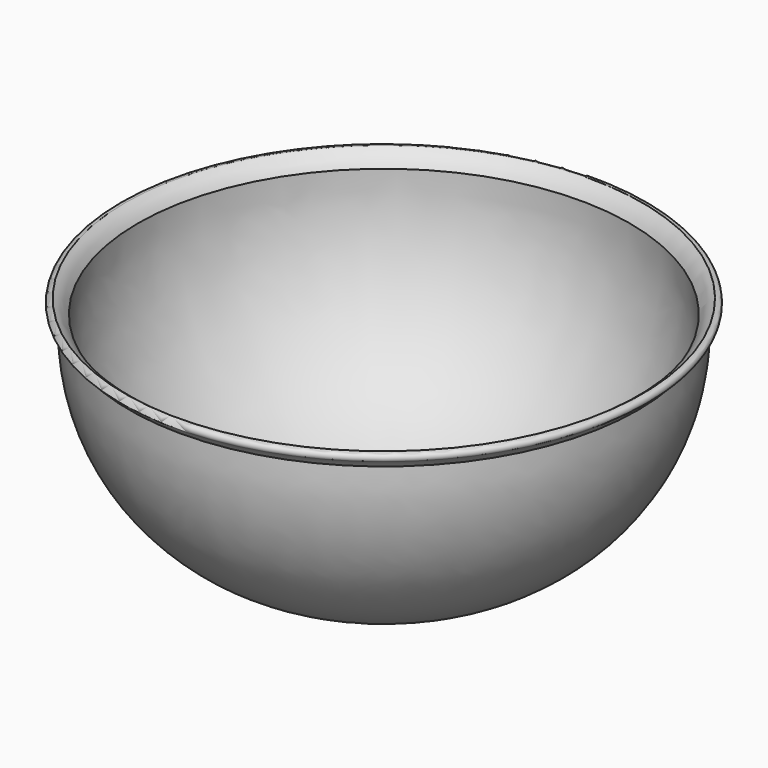
from build123d import *

# Parameters (mm, degrees)
F2_TEXT_SIZE = 18.1491480261
F3_DEPTH     = 3.175


# Not quite as in the source:
# - Text() gives the source's letters only with a copy of the font that has no kerning and outlines rounded to 1/6400 em; it was checked with that copy


with BuildPart() as f1:
    # F0 (on Front) → F1 (revolve)
    with BuildSketch(Plane.XZ):
        with BuildLine():
            ThreePointArc((0, 0), (-34.2352394172, 31.1750034287), (-45.0371901893, 76.2))
            ThreePointArc((-45.0371901893, 76.2), (-47.0998938701, 79.2854492393), (-49.9665268701, 81.6428119026))
            ThreePointArc((-49.9665268701, 81.6428119026), (-51.8145206739, 80.9019000279), (-51.6031930226, 78.9221596084))
            ThreePointArc((-51.6031930226, 78.9221596084), (-49.7126642737, 77.4294196755), (-48.2570643, 75.5101489353))
            ThreePointArc((-48.2570643, 75.5101489353), (-36.5560461644, 28.8693888765), (-0.7031318367, -3.175))
            Line((-0.7031318367, -3.175), (50.8, -3.175))
            Line((50.8, -3.175), (50.8, 0))
            Line((50.8, 0), (0, 0))
        make_face()
    revolve(axis=Axis((50.8, 0, -1.5875), (0, 0, 1)))

    # F2 (on face) → F3 (join)
    with BuildSketch(Plane.XY):
        with Locations((19.6840073913, -6.253677886)):
            Text('FILL ME', F2_TEXT_SIZE, font='Open Sans', font_style=FontStyle.BOLD, text_align=(TextAlign.LEFT, TextAlign.BOTTOM))
    extrude(amount=F3_DEPTH)


solid = f1.part
